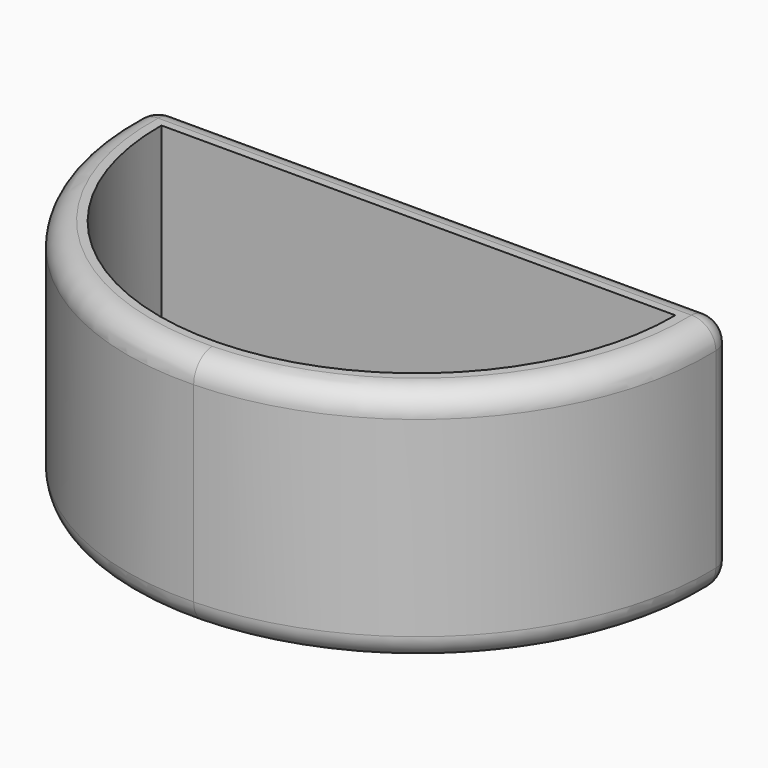
from build123d import *

# Parameters (mm, degrees)
F1_DEPTH = 30
F3_R     = 3


# Not quite as in the source:
# - a feature of the source that left no trace in its solid (it failed there, or was rolled back) is left out


with BuildPart() as f1:
    # F0 (on Top) → F1 (new body)
    with BuildSketch(Plane.XY):
        with BuildLine():
            ThreePointArc((-37.25, 36.5), (-27.8459144936, 7.7690354349), (0, -4))
            ThreePointArc((0, -4), (26.5127811208, 8.5143386541), (35.25, 36.5))
            Line((35.25, 36.5), (-37.25, 36.5))
        make_face()
        with BuildLine():
            ThreePointArc((0, 0), (-23.5433609961, 9.1719845194), (-33.25, 32.5))
            Line((-33.25, 32.5), (31.25, 32.5))
            ThreePointArc((31.25, 32.5), (22.2476477305, 9.8820694899), (0, 0))
        make_face(mode=Mode.SUBTRACT)
    extrude(amount=F1_DEPTH)

    # F3
    f3_edges = [f1.edges().sort_by_distance(p)[0] for p in [
        (-1, 36.5, 0),
        (-1, -4.013711, 0),
        (-37.25, 36.5, 15),
        (35.25, 36.5, 15),
        (-1, 36.5, 30),
        (-1, -4.013711, 30),
    ]]
    fillet(f3_edges, radius=F3_R)


solid = f1.part
